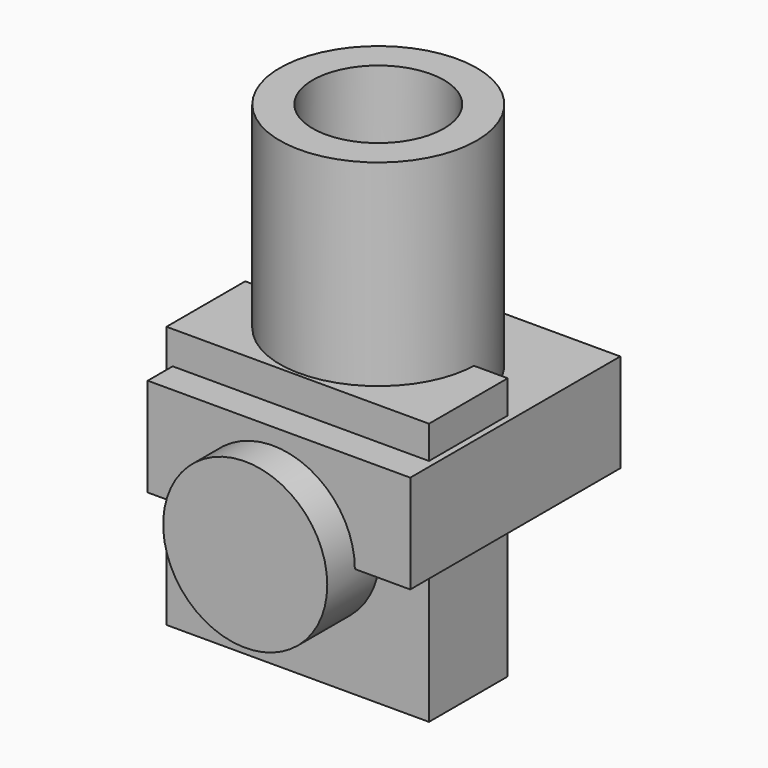
from build123d import *

# Parameters (mm, degrees)
F0_W     = 8
F0_H     = 8
F1_DEPTH = 3
F2_R     = 2.5
F3_DEPTH = 5
F4_W     = 8
F4_H     = 8
F5_DEPTH = 3
F6_R     = 3
F6_R_2   = 2
F7_DEPTH = 10


with BuildPart() as f1:
    # F0 (on Front) → F1 (new body)
    with BuildSketch(Plane.XZ):
        Rectangle(F0_W, F0_H)
    extrude(amount=F1_DEPTH)

    # F2 (on Front) → F3 (join)
    with BuildSketch(Plane.XZ):
        Circle(F2_R)
    extrude(amount=F3_DEPTH)


with BuildPart() as f5:
    # F4 (on Top) → F5 (new body)
    with BuildSketch(Plane.XY):
        with Locations((0.1882740475, 0.0510183199)):
            Rectangle(F4_W, F4_H)
    extrude(amount=F5_DEPTH)

    # F6 (on Top) → F7 (join)
    with BuildSketch(Plane.XY):
        with Locations((-0.0257475294, 0.1019836782)):
            Circle(F6_R)
        with Locations((-0.0257475294, 0.1019836782)):
            Circle(F6_R_2, mode=Mode.SUBTRACT)
    extrude(amount=F7_DEPTH)


solid = Compound([f1.part, f5.part])
